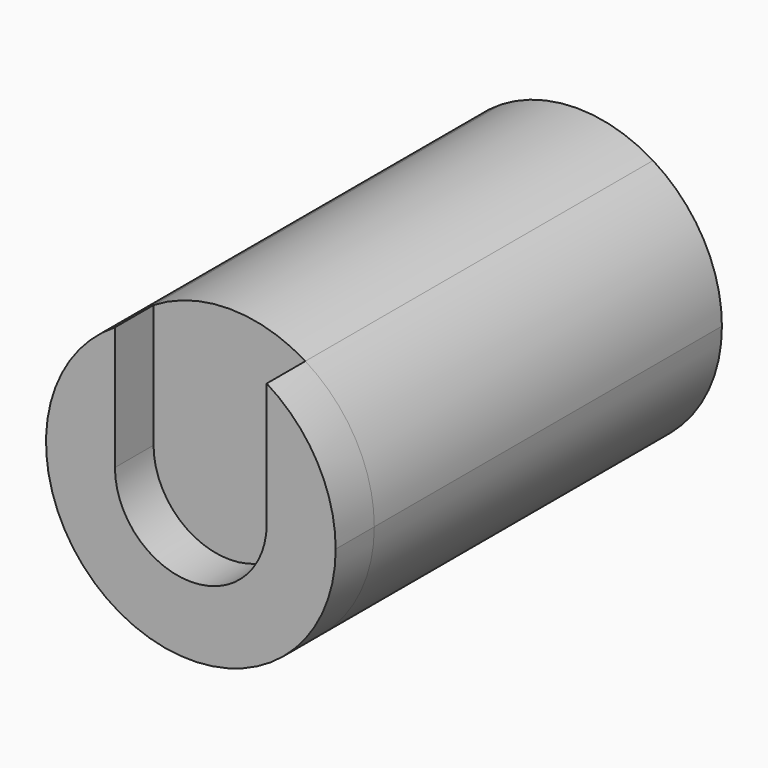
from build123d import *
from build123d import SkipClean  # not in build123d's __all__

# Parameters (mm, degrees)
F1_DEPTH = 5
F2_R     = 1.5
F3_DEPTH = 4.5


with BuildPart() as f1:
    # F0 (on Front) → F1 (new body)
    with BuildSketch(Plane.XZ):
        with BuildLine():
            ThreePointArc((-0.786, 1.2775773949), (-0.7317786551, -1.3093891706), (1.5, 0))
            ThreePointArc((1.5, 0), (1.3093891706, 0.7317786551), (0.786, 1.2775773949))
            Line((0.786, 1.2775773949), (0.786, 0))
            ThreePointArc((0.786, 0), (0, -0.786), (-0.786, 0))
            Line((-0.786, 0), (-0.786, 1.2775773949))
        make_face()
    extrude(amount=F1_DEPTH)

    # F2 (on face) → F3 (join)
    with BuildSketch(Plane(origin=(0, 0, 0), x_dir=(-1, 0, 0), z_dir=(0, 1, 0))):
        Circle(F2_R)
    with SkipClean():  # cleaning this boolean's faces spoils the solid; the shape is the same uncleaned
        extrude(amount=-F3_DEPTH)


solid = f1.part
